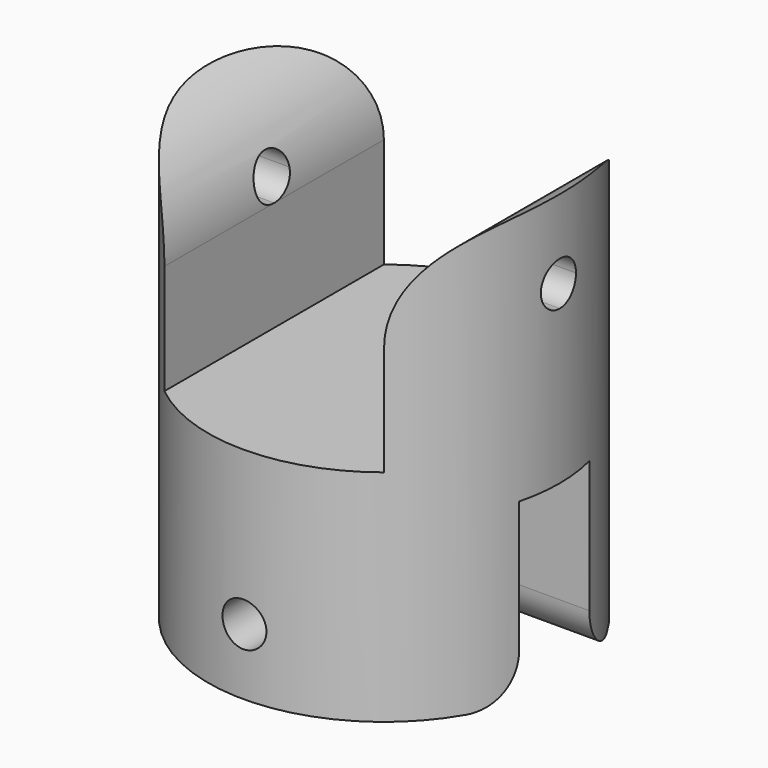
from build123d import *

# Parameters (mm, degrees)
F0_R        = 8
F1_DEPTH    = 10
F3_DEPTH    = 10
F5_DEPTH    = 8
F6_R        = 2
F7_T1_DEPTH = 37.4899959968
F9_DEPTH    = 12.5
F11_DEPTH   = 12.5


# Not quite as in the source:
# - a fillet or chamfer that OpenCascade refuses, or shapes differently, is made with other operations: its cross-section is extruded or revolved along the edge and cut away or added


with BuildPart() as f1:
    # F0 (on Top) → F1 (new body, symmetric)
    with BuildSketch(Plane.XY):
        Circle(F0_R)
    extrude(amount=F1_DEPTH, both=True)

    # F2 (on face) → F3 (cut)
    with BuildSketch(Plane.XY.offset(10)):
        with BuildLine():
            ThreePointArc((5, 6.2449979984), (0, 8), (-5, 6.2449979984))
            Line((-5, 6.2449979984), (-5, -6.2449979984))
            ThreePointArc((-5, -6.2449979984), (0, -8), (5, -6.2449979984))
            Line((5, -6.2449979984), (5, 6.2449979984))
        make_face()
    extrude(amount=-F3_DEPTH, mode=Mode.SUBTRACT)

    # F4 (on face) → F5 (cut)
    with BuildSketch(Plane(origin=(0, 0, -10), x_dir=(1, 0, 0), z_dir=(0, 0, -1))):
        with BuildLine():
            Line((7.7459666924, 2), (-7.7459666924, 2))
            ThreePointArc((-7.7459666924, 2), (-8, 0), (-7.7459666924, -2))
            Line((-7.7459666924, -2), (7.7459666924, -2))
            ThreePointArc((7.7459666924, -2), (7.9362375701, -1.0080343399), (8, 0))
            ThreePointArc((8, 0), (7.9362375701, 1.0080343399), (7.7459666924, 2))
        make_face()
    extrude(amount=-F5_DEPTH, mode=Mode.SUBTRACT)

    # F6
    f6_edges = [f1.edges().sort_by_distance(p)[0] for p in [
        (0, 2, -10),
        (0, -2, -10),
    ]]
    fillet(f6_edges, radius=F6_R)

    # F7: fillet of radius 5 on 2 edges, made by hand

    # F7_s2 → F7_t1 (cut)
    with BuildSketch(Plane.XZ.offset(-18.7449979984)):
        with BuildLine():
            ThreePointArc((-5, 5), (-6.4644660941, 8.5355339059), (-10, 10))
            Line((-10, 10), (-5, 10))
            Line((-5, 10), (-5, 5))
        make_face()
        with BuildLine():
            ThreePointArc((10, 10), (6.4644660941, 8.5355339059), (5, 5))
            Line((5, 5), (5, 10))
            Line((5, 10), (10, 10))
        make_face()
    extrude(amount=F7_T1_DEPTH, mode=Mode.SUBTRACT)

    # F8 (on Right) → F9 (cut, symmetric)
    with BuildSketch(Plane.YZ):
        with BuildLine():
            ThreePointArc((0, 5), (0.7071067812, 5.2928932188), (1, 6))
            ThreePointArc((1, 6), (-0.7071067812, 6.7071067812), (0, 5))
        make_face()
    extrude(amount=F9_DEPTH, both=True, mode=Mode.SUBTRACT)

    # F10 (on Front) → F11 (cut, symmetric)
    with BuildSketch(Plane.XZ):
        with BuildLine():
            ThreePointArc((0, -6), (-0.7071067812, -7.7071067812), (1, -7))
            ThreePointArc((1, -7), (0.7071067812, -6.2928932188), (0, -6))
        make_face()
    extrude(amount=F11_DEPTH, both=True, mode=Mode.SUBTRACT)


solid = f1.part
